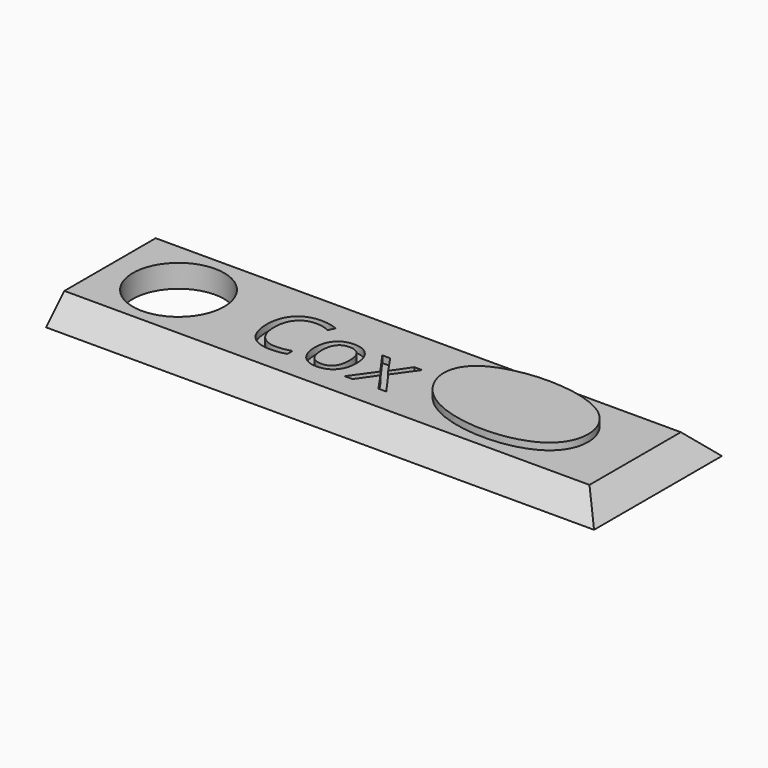
from build123d import *

# Parameters (mm, degrees)
F0_W         = 120
F0_H         = 35
F0_R         = 10
F1_DEPTH     = 5
F2_SIZE      = 4.99999
F3_TEXT_SIZE = 18.7931181346
F4_DEPTH     = 1.5
F6_DEPTH     = 1.5


# Not quite as in the source:
# - a fillet or chamfer is up to 0.001 mm smaller than in the source, because OpenCascade refuses the exact size
# - Text() gives the source's letters only with a copy of the font that has no kerning and outlines rounded to 1/6400 em; it was checked with that copy


with BuildPart() as f1:
    # F0 (on Top) → F1 (new body)
    with BuildSketch(Plane.XY):
        Rectangle(F0_W, F0_H)
        with Locations((-45, 0)):
            Circle(F0_R, mode=Mode.SUBTRACT)
    extrude(amount=F1_DEPTH)

    # F2 (size 5 in the source; OpenCascade refuses exactly that, so slightly less here)
    f2_edges = [f1.edges().sort_by_distance(p)[0] for p in [
        (0, 17.5, 5),
        (0, -17.5, 5),
        (60, 0, 5),
    ]]
    chamfer(f2_edges, length=F2_SIZE)

    # F3 (on face) → F4 (cut)
    with BuildSketch(Plane.XY.offset(5)):
        with Locations((-26.4048464596, -7.2165569291)):
            Text('Cox', F3_TEXT_SIZE, font='Open Sans', text_align=(TextAlign.LEFT, TextAlign.BOTTOM))
    extrude(amount=-F4_DEPTH, mode=Mode.SUBTRACT)

    # F5 (on face) → F6 (join)
    with BuildSketch(Plane.XY.offset(5)):
        with BuildLine():
            add(Edge.make_bspline(
                [(13.3223673329, 6.8092108704), (18.3725870455, 12.0604248929), (45.0023778462, 12.8007586384), (46.8617892522, -11.2284919271), (13.7833015726, -11.3673846598), (9.7584632039, 3.1034664867), (13.3223673329, 6.8092108704)],
                knots=[0, 0, 0, 0, 0.2960245185, 0.5048051202, 0.7910976029, 1, 1, 1, 1], degree=3))
        make_face()
    extrude(amount=F6_DEPTH)


solid = f1.part
